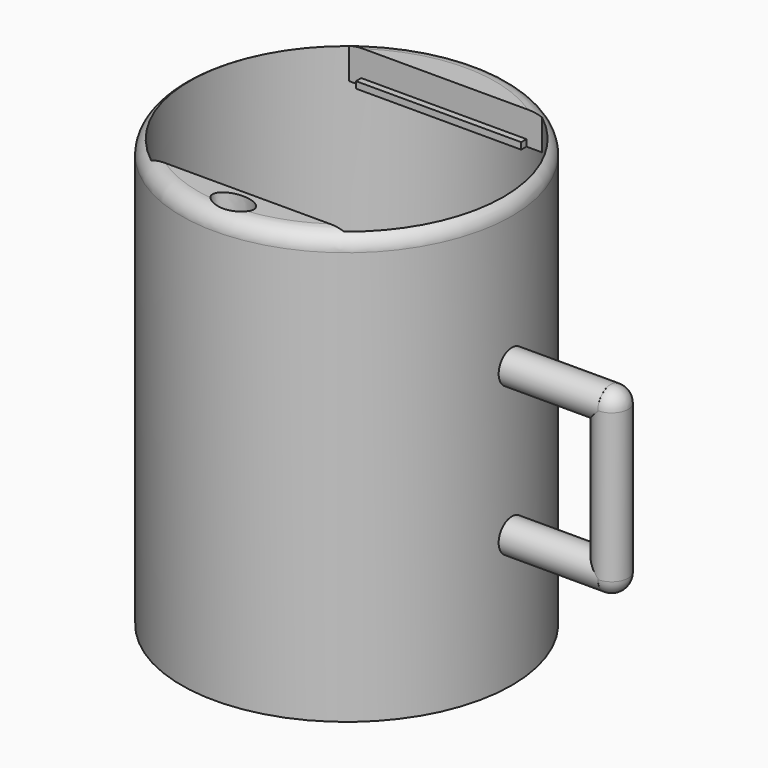
from build123d import *

# Parameters (mm, degrees)
F0_R      = 50
F1_DEPTH  = 130
F2_R      = 47.5
F3_DEPTH  = 90
F5_DEPTH  = 10
F7_DEPTH  = 10
F9_DEPTH  = 10
F10_W     = 50
F10_H     = 2
F11_DEPTH = 2
F14_R     = 5
F15_DEPTH = 30
F20_R     = 5
F21_DEPTH = 55
F22_R     = 5
F18_R     = 5
F23_DEPTH = 25
F24_W     = 50
F24_H     = 2
F25_DEPTH = 2
F26_R     = 2.5
F27_DEPTH = 60


# Not quite as in the source:
# - a fillet or chamfer that OpenCascade refuses, or shapes differently, is made with other operations: its cross-section is extruded or revolved along the edge and cut away or added


with BuildPart() as f1:
    # F0 (on Top) → F1 (new body)
    with BuildSketch(Plane.XY):
        Circle(F0_R)
    extrude(amount=F1_DEPTH)

    # F2 (on face) → F3 (cut)
    with BuildSketch(Plane.XY.offset(130)):
        Circle(F2_R)
    extrude(amount=-F3_DEPTH, mode=Mode.SUBTRACT)

    # F4 (on face) → F5 (join)
    with BuildSketch(Plane.XY.offset(130)):
        with BuildLine():
            Line((29.2207095994, -37.4486332262), (-29.2207095994, -37.4486332262))
            ThreePointArc((-29.2207095994, -37.4486332262), (0, -47.5), (29.2207095994, -37.4486332262))
        make_face()
    extrude(amount=-F5_DEPTH)

    # F6 (on face) → F7 (cut)
    with BuildSketch(Plane.XY.offset(130)):
        with BuildLine():
            add(Edge.make_bspline(
                [(-6.25, -42.9242551327), (-6.25, -49.4194456611), (3.125, -46.1718503969), (12.5, -42.9242551327), (3.125, -39.6766598685), (-6.25, -36.4290646043), (-6.25, -42.9242551327)],
                knots=[0, 0, 0, 2.0943951024, 2.0943951024, 4.1887902048, 4.1887902048, 6.2831853072, 6.2831853072, 6.2831853072], degree=2, weights=[1, 0.5, 1, 0.5, 1, 0.5, 1]))
        make_face()
    extrude(amount=-F7_DEPTH, mode=Mode.SUBTRACT)

    # F8 (on face) → F9 (join)
    with BuildSketch(Plane.XY.offset(130)):
        with BuildLine():
            ThreePointArc((29.22, 37.4491869071), (0, 47.5), (-29.22, 37.4491869071))
            Line((-29.22, 37.4491869071), (29.22, 37.4491869071))
        make_face()
    extrude(amount=-F9_DEPTH)

    # F10 (on face) → F11 (join)
    with BuildSketch(Plane.XZ.offset(-37.4491869071)):
        with Locations((-0.5380645394, 121)):
            Rectangle(F10_W, F10_H)
    extrude(amount=F11_DEPTH)

    # F12: fillet of radius 5 on 1 edges, made by hand

    # F12_s1 → F12_t2 (revolve, cut)
    with BuildSketch(Plane.XZ):
        with BuildLine():
            ThreePointArc((50, 125), (48.5355339059, 128.5355339059), (45, 130))
            Line((45, 130), (50, 130))
            Line((50, 130), (50, 125))
        make_face()
    revolve(axis=Axis((0, 0, 130), (0, 0, 1)), mode=Mode.SUBTRACT)

    # F18 (on offset) → F23 (cut)
    with BuildSketch(Plane.YZ.offset(-50)):
        with Locations((0, 55)):
            Circle(F18_R)
    extrude(amount=F23_DEPTH, mode=Mode.SUBTRACT)

    # F24 (on face) → F25 (join)
    with BuildSketch(Plane(origin=(0, -37.4486332262, 0), x_dir=(-1, 0, 0), z_dir=(0, 1, 0))):
        with Locations((-1.0655004531, 121)):
            Rectangle(F24_W, F24_H)
    extrude(amount=F25_DEPTH)

    # F26 (on face) → F27 (join)
    with BuildSketch(Plane.XY.offset(40)):
        Circle(F26_R)
    extrude(amount=F27_DEPTH)


with BuildPart() as f15:
    # F14 (on offset) → F15 (new body)
    with BuildSketch(Plane.YZ.offset(50)):
        with Locations((0, 85)):
            Circle(F14_R)
    extrude(amount=F15_DEPTH)


with BuildPart() as f15b:
    # F14 (on offset) → F15, piece 2 (new body)
    with BuildSketch(Plane.YZ.offset(50)):
        with Locations((0, 40)):
            Circle(F14_R)
    extrude(amount=F15_DEPTH)


with BuildPart() as f21:
    # F20 (on offset) → F21 (new body)
    with BuildSketch(Plane.XY.offset(90)):
        with Locations((80.2221212434, 0)):
            Circle(F20_R)
    extrude(amount=-F21_DEPTH)

    # F22
    f22_edges = [f21.edges().sort_by_distance(p)[0] for p in [
        (75.222121, 0, 35),
        (75.222121, 0, 90),
        (85.222121, 0, 62.5),
    ]]
    fillet(f22_edges, radius=F22_R)


solid = Compound([f1.part, f15.part, f15b.part, f21.part])
